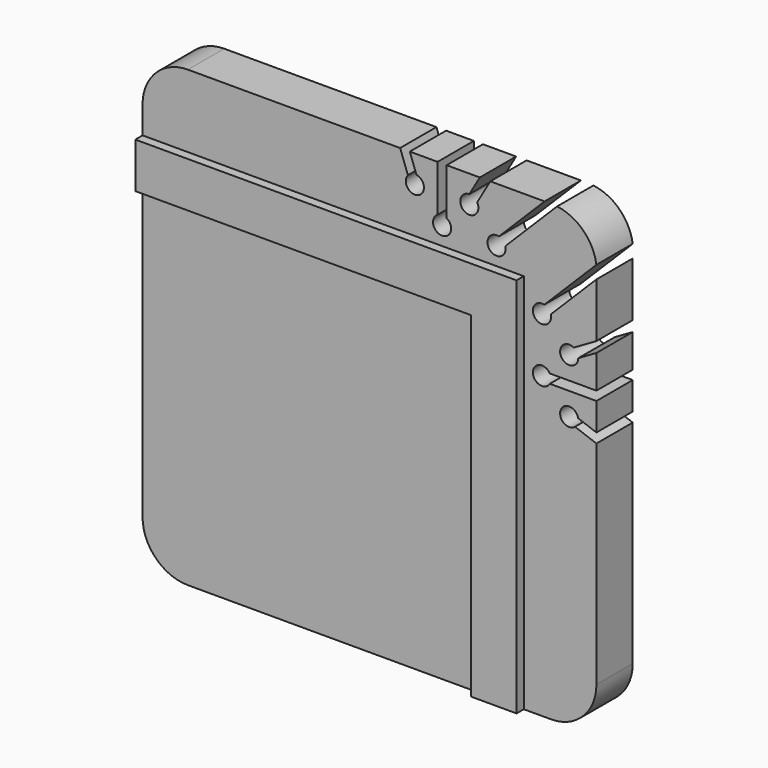
from build123d import *

# Parameters (mm, degrees)
F2_DEPTH    = 5
F3_DEPTH    = 1
F4_DEPTH    = 5
F7_T1_DEPTH = 29.7487373415
F7_T3_DEPTH = 30


# Not quite as in the source:
# - a fillet or chamfer that OpenCascade refuses, or shapes differently, is made with other operations: its cross-section is extruded or revolved along the edge and cut away or added


with BuildPart() as f2:
    # F0 (on Front) → F2 (new body)
    with BuildSketch(Plane.XZ):
        Polygon((0, 37), (0, 0), (37, 37), align=None)
        Polygon((0, 42), (0, 37), (37, 37), (42, 42), align=None)
        Polygon((42, 42), (50, 50), (0, 50), (0, 42), align=None)
    extrude(amount=-F2_DEPTH)

    # F1 (on Front) → F4 (cut, through all)
    with BuildSketch(Plane.XZ):
        with BuildLine():
            ThreePointArc((29.2339555569, 47.6427876097), (29.6579798567, 46.0603073792), (31, 47))
            ThreePointArc((31, 47), (30.7660444431, 47.6427876097), (30.1736481777, 47.984807753))
            ThreePointArc((30.1736481777, 47.984807753), (29.6579798567, 47.9396926208), (29.2339555569, 47.6427876097))
        make_face()
        with BuildLine():
            ThreePointArc((29.2339555569, 47.6427876097), (29.6579798567, 47.9396926208), (30.1736481777, 47.984807753))
            Line((30.1736481777, 47.984807753), (29.4401781834, 50))
            Line((29.4401781834, 50), (28.376000411, 50))
            Line((28.376000411, 50), (29.2339555569, 47.6427876097))
        make_face()
        with BuildLine():
            ThreePointArc((32.5, 44.8660254038), (32.5, 43.1339745962), (34, 44))
            ThreePointArc((34, 44), (33.8660254038, 44.5), (33.5, 44.8660254038))
            ThreePointArc((33.5, 44.8660254038), (33, 45), (32.5, 44.8660254038))
        make_face()
        with BuildLine():
            ThreePointArc((32.5, 44.8660254038), (33, 45), (33.5, 44.8660254038))
            Line((33.5, 44.8660254038), (33.5, 50))
            Line((33.5, 50), (32.5, 50))
            Line((32.5, 50), (32.5, 44.8660254038))
        make_face()
        with BuildLine():
            ThreePointArc((36, 48), (35.2928932188, 46.2928932188), (37, 47))
            ThreePointArc((37, 47), (36.9659258263, 47.2588190451), (36.8660254038, 47.5))
            ThreePointArc((36.8660254038, 47.5), (36.5, 47.8660254038), (36, 48))
        make_face()
        with BuildLine():
            ThreePointArc((39.2588190451, 44.9659258263), (38.2066466597, 43.391238571), (40, 44))
            ThreePointArc((40, 44), (39.9914448614, 44.1305261922), (39.9659258263, 44.2588190451))
            ThreePointArc((39.9659258263, 44.2588190451), (39.7071067812, 44.7071067812), (39.2588190451, 44.9659258263))
        make_face()
        with BuildLine():
            ThreePointArc((39.2588190451, 44.9659258263), (39.7071067812, 44.7071067812), (39.9659258263, 44.2588190451))
            Line((39.9659258263, 44.2588190451), (45.7071067812, 50))
            Line((45.7071067812, 50), (44.2928932188, 50))
            Line((44.2928932188, 50), (39.2588190451, 44.9659258263))
        make_face()
        with BuildLine():
            ThreePointArc((36, 48), (36.5, 47.8660254038), (36.8660254038, 47.5))
            Line((36.8660254038, 47.5), (38.3094010768, 50))
            Line((38.3094010768, 50), (37.1547005384, 50))
            Line((37.1547005384, 50), (36, 48))
        make_face()
    extrude(amount=-F4_DEPTH, mode=Mode.SUBTRACT)

    # F5: F2 across face


with BuildPart() as f3:
    # F0 (on Front) → F3 (new body)
    with BuildSketch(Plane.XZ):
        Polygon((0, 42), (0, 37), (37, 37), (42, 42), align=None)
    extrude(amount=F3_DEPTH)

    # F6: F3 across face


with BuildPart() as f2_1:
    add(f2.part)
    add(f2.part.mirror(Plane(origin=(25, 2.5, 25), x_dir=(0, 1, 0), z_dir=(0.7071067812, 0, -0.7071067812))))

    # F7: fillet of radius 5 on 4 edges, made by hand

    # F7_s2 → F7_t1 (cut)
    with BuildSketch(Plane.XZ.offset(-17.3743686708)):
        with BuildLine():
            ThreePointArc((45.0502525317, 50), (48.3262612385, 48.777269775), (50, 45.7071067812))
            Line((50, 45.7071067812), (50, 50))
            Line((50, 50), (45.0502525317, 50))
        make_face()
    extrude(amount=F7_T1_DEPTH, mode=Mode.SUBTRACT)

    # F7_s4 → F7_t3 (cut)
    with BuildSketch(Plane.XZ.offset(-17.5)):
        with BuildLine():
            ThreePointArc((0, 5), (1.4644660941, 1.4644660941), (5, 0))
            Line((5, 0), (0, 0))
            Line((0, 0), (0, 5))
        make_face()
        with BuildLine():
            ThreePointArc((45, 0), (48.5355339059, 1.4644660941), (50, 5))
            Line((50, 5), (50, 0))
            Line((50, 0), (45, 0))
        make_face()
        with BuildLine():
            ThreePointArc((0, 45), (1.4644660941, 48.5355339059), (5, 50))
            Line((5, 50), (0, 50))
            Line((0, 50), (0, 45))
        make_face()
    extrude(amount=F7_T3_DEPTH, mode=Mode.SUBTRACT)


with BuildPart() as f3_1:
    add(f3.part)
    add(f3.part.mirror(Plane(origin=(39.5, -0.5, 39.5), x_dir=(0, 1, 0), z_dir=(0.7071067812, 0, -0.7071067812))))


solid = Compound([f2_1.part, f3_1.part])
